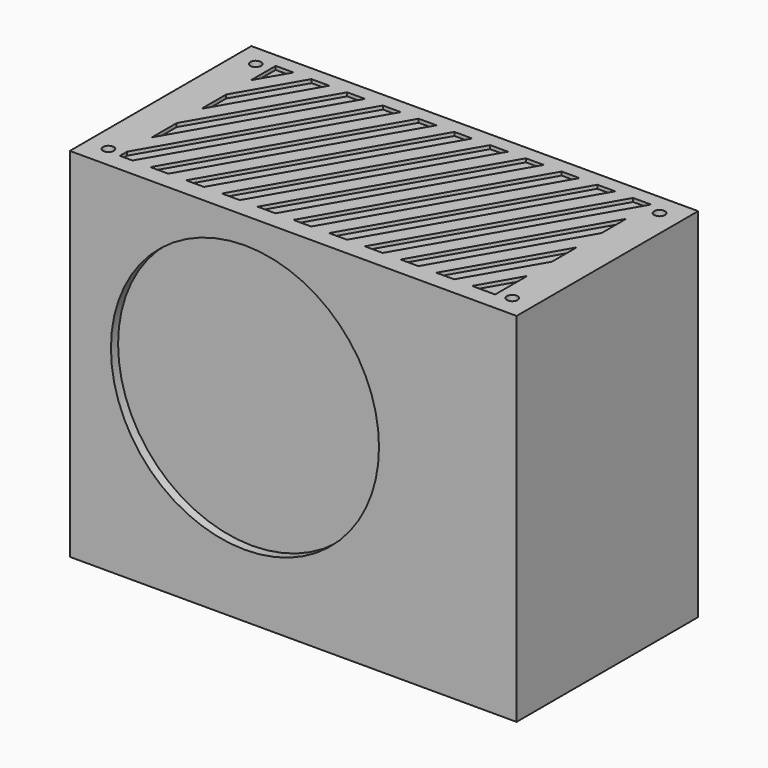
from build123d import *

# Parameters (mm, degrees)
F0_W     = 125
F0_H     = 100
F2_DEPTH = 63.5
F1_R     = 37.5
F3_DEPTH = 2.5
F5_DEPTH = 1
F6_R     = 1.5
F7_DEPTH = 20


# Not quite as in the source:
# - a feature names something its author has since deleted; it is built from what else it names


with BuildPart() as f2:
    # F0 (on Front) → F2 (new body)
    with BuildSketch(Plane.XZ):
        with Locations((0, 17.5)):
            Rectangle(F0_W, F0_H)
    extrude(amount=-F2_DEPTH)

    # F1 (on Front) → F3 (cut, symmetric)
    with BuildSketch(Plane.XZ):
        with Locations((-13.5, 22.6666666667)):
            Circle(F1_R)
    extrude(amount=F3_DEPTH, both=True, mode=Mode.SUBTRACT)

    # F4 (on face) → F5 (cut)
    with BuildSketch(Plane.XY.offset(67.5)):
        Polygon((51.0344103292, 5), (52.5, 5), (52.5, 7.5384757729), align=None)
        Polygon((46.0344103292, 5), (51.0344103292, 5), (52.5, 7.5384757729), (52.5, 16.1987298108), align=None)
        Polygon((36.0344103292, 5), (41.0344103292, 5), (52.5, 24.8589838486), (52.5, 33.5192378865), align=None)
        Polygon((26.0344103292, 5), (31.0344103292, 5), (52.5, 42.1794919243), (52.5, 50.8397459622), align=None)
        Polygon((16.0344103292, 5), (21.0344103292, 5), (52.5, 59.5), (47.5, 59.5), align=None)
        Polygon((-32.5, 59.5), (-52.5, 24.8589838486), (-52.5, 16.1987298108), (-27.5, 59.5), align=None)
        Polygon((6.0344103292, 5), (11.0344103292, 5), (42.5, 59.5), (37.5, 59.5), align=None)
        Polygon((-52.5, 42.1794919243), (-52.5, 33.5192378865), (-37.5, 59.5), (-42.5, 59.5), align=None)
        Polygon((-47.5, 59.5), (-52.5, 59.5), (-52.5, 50.8397459622), align=None)
        Polygon((-22.5, 59.5), (-52.5, 7.5384757729), (-52.5, 5), (-48.9655896708, 5), (-17.5, 59.5), align=None)
        Polygon((-3.9655896708, 5), (1.0344103292, 5), (32.5, 59.5), (27.5, 59.5), align=None)
        Polygon((-13.9655896708, 5), (-8.9655896708, 5), (22.5, 59.5), (17.5, 59.5), align=None)
        Polygon((-12.5, 59.5), (-43.9655896708, 5), (-38.9655896708, 5), (-7.5, 59.5), align=None)
        Polygon((-23.9655896708, 5), (-18.9655896708, 5), (12.5, 59.5), (7.5, 59.5), align=None)
        Polygon((-2.5, 59.5), (-33.9655896708, 5), (-28.9655896708, 5), (2.5, 59.5), align=None)
    extrude(amount=-F5_DEPTH, mode=Mode.SUBTRACT)

    # F6 (on face) → F7 (cut)
    with BuildSketch(Plane.XY.offset(67.5)):
        with Locations((-56.5, 57.5)):
            Circle(F6_R)
        with Locations((56.5, 57.5)):
            Circle(F6_R)
        with Locations((56.5, 6)):
            Circle(F6_R)
        with Locations((-56.5, 6)):
            Circle(F6_R)
    extrude(amount=-F7_DEPTH, mode=Mode.SUBTRACT)


solid = f2.part
